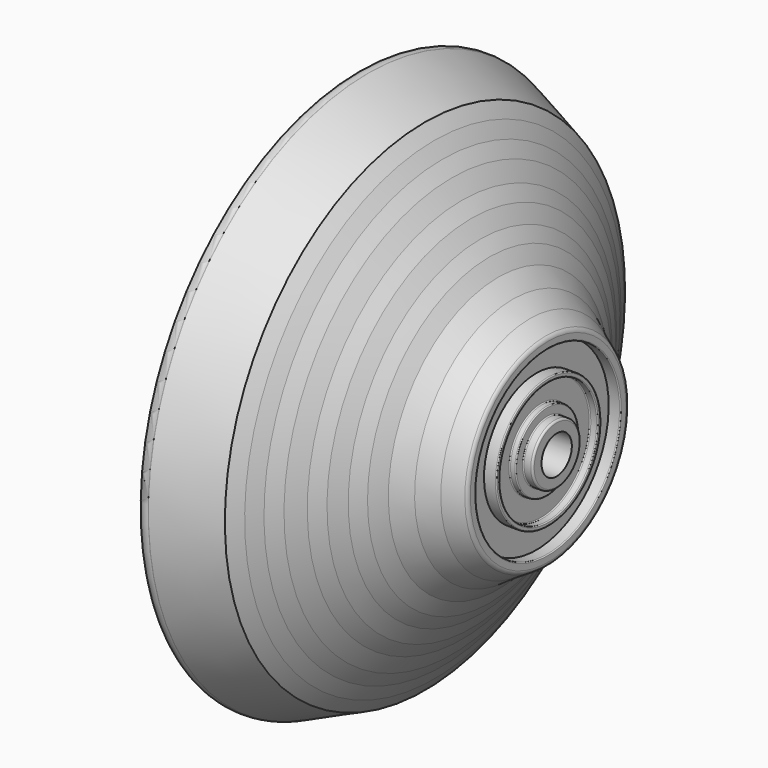
from build123d import *

# Parameters (mm, degrees)
F2_R = 0.1
F3_R = 0.2
F4_R = 0.5
F5_R = 0.5
F8_R = 0.85


with BuildPart() as f1:
    # F0 (on Front) → F1 (revolve)
    with BuildSketch(Plane.XZ):
        with BuildLine():
            Line((-4.2, 2), (-1.4, 2))
            Line((-1.4, 2), (-1.4, 3.17))
            Line((-1.4, 3.17), (-2.4, 3.17))
            Line((-2.4, 3.17), (-2.4, 4.15))
            Line((-2.4, 4.15), (-3.05, 4.15))
            Line((-3.05, 4.15), (-3.05, 6.45))
            Line((-3.05, 6.45), (-2.25, 6.45))
            Line((-2.25, 6.45), (-2.25, 6.9))
            Line((-2.25, 6.9), (-3.55, 6.9))
            Line((-3.55, 6.9), (-3.55, 9.55))
            Line((-3.55, 9.55), (-2.3, 9.55))
            Line((-2.3, 9.55), (-2.3, 10.55))
            Line((-2.3, 10.55), (-4.2488235049, 11.7284217849))
            Line((-4.2488235049, 11.7284217849), (-6.0193808361, 12.9681793751))
            Line((-6.0193808361, 12.9681793751), (-7.5602556007, 14.5090541396))
            Line((-7.5602556007, 14.5090541396), (-9.4593313096, 17.4266965415))
            Line((-9.4593313096, 17.4266965415), (-11.397791514, 20.4048472599))
            Line((-11.397791514, 20.4048472599), (-13.4484577999, 23.5553856402))
            Line((-13.4484577999, 23.5553856402), (-15.2898428789, 26.3843951207))
            Line((-15.2898428789, 26.3843951207), (-15.3, 26.4))
            Line((-15.3, 26.4), (-21.3, 26.4))
            Line((-21.3, 26.4), (-21.3, 28.9833333333))
            Line((-21.3, 28.9833333333), (-22.5, 29.5))
            Line((-22.5, 29.5), (-22.5, 24.5013962977))
            ThreePointArc((-22.5, 24.5013962977), (-21.9482556511, 23.6074908938), (-20.9018662575, 23.7))
            Line((-20.9018662575, 23.7), (-20.5080900341, 24.4))
            Line((-20.5080900341, 24.4), (-15.4300203026, 24.4))
            Line((-15.4300203026, 24.4), (-14.8718719174, 23.5424894817))
            Line((-14.8718719174, 23.5424894817), (-13.0431798353, 20.7329808699))
            Line((-13.0431798353, 20.7329808699), (-11.1785135129, 17.8682032825))
            Line((-11.1785135129, 17.8682032825), (-9.4125806174, 15.1551146623))
            Line((-9.4125806174, 15.1551146623), (-8.5412627086, 13.8106271625))
            Line((-8.5412627086, 13.8106271625), (-8.0127408728, 12.4712157995))
            Line((-8.0127408728, 12.4712157995), (-7.6767695136, 11.0429953784))
            Line((-7.6767695136, 11.0429953784), (-7.5, 9.6929371357))
            Line((-7.5, 9.6929371357), (-7.5, 8.5))
            Line((-7.5, 8.5), (-4.75, 8.5))
            Line((-4.75, 8.5), (-4.8163929872, 7.8235659748))
            Line((-4.8163929872, 7.8235659748), (-4.75, 7.1570291184))
            Line((-4.75, 7.1570291184), (-4.8163929872, 6.4776679501))
            Line((-4.8163929872, 6.4776679501), (-4.75, 5.7739662006))
            Line((-4.75, 5.7739662006), (-4.25, 5.7739662006))
            Line((-4.25, 5.7739662006), (-4.3176623901, 5.0816159641))
            Line((-4.3176623901, 5.0816159641), (-4.25, 4.4365157373))
            Line((-4.25, 4.4365157373), (-4.3095897044, 3.8267686403))
            Line((-4.3095897044, 3.8267686403), (-4.25, 3.17))
            Line((-4.25, 3.17), (-4.9999979152, 2.6389400014))
            Line((-4.9999979152, 2.6389400014), (-5.4533858784, 1.9280725392))
            Line((-5.4533858784, 1.9280725392), (-5.7284533243, 1.1602115126))
            Line((-5.7284533243, 1.1602115126), (-6.078645587, 0.5922464188))
            Line((-6.078645587, 0.5922464188), (-6.3, 0))
            Line((-6.3, 0), (-5.1852456548, 0))
            Line((-5.1852456548, 0), (-4.2, 2))
        make_face()
        Polygon((-9.4593313096, 17.4266965415), (-7.5602556007, 14.5090541396), (-8.4929022586, 16.0905005494), align=None)
        Polygon((-11.397791514, 20.4048472599), (-9.4593313096, 17.4266965415), (-10.4045527072, 19.0459996231), align=None)
        Polygon((-13.4484577999, 23.5553856402), (-11.397791514, 20.4048472599), (-12.4549735292, 22.1575423946), align=None)
        Polygon((-15.2898428789, 26.3843951207), (-13.4484577999, 23.5553856402), (-14.3121259439, 25.0234248466), align=None)
        Polygon((-10.3353289936, 16.4669086803), (-9.4125806174, 15.1551146623), (-11.1785135129, 17.8682032825), align=None)
        Polygon((-12.1445821899, 19.2208318679), (-11.1785135129, 17.8682032825), (-13.0431798353, 20.7329808699), align=None)
        Polygon((-14.0160004839, 22.095063141), (-13.0431798353, 20.7329808699), (-14.8718719174, 23.5424894817), align=None)
    revolve(axis=Axis((-5.7426228274, 0, 0), (-1, 0, 0)))

    # F2
    f2_edges = [f1.edges().sort_by_distance(p)[0] for p in [
        (-2.4, 0, -4.15),
        (-3.05, 0, -4.15),
        (-2.25, 0, -6.45),
        (-2.25, 0, -6.9),
        (-2.3, 0, -9.55),
        (-3.05, 0, -6.45),
        (-2.4, 0, -3.17),
    ]]
    fillet(f2_edges, radius=F2_R)

    # F3
    f3_edges = [f1.edges().sort_by_distance(p)[0] for p in [
        (-1.4, 0, -3.17),
    ]]
    fillet(f3_edges, radius=F3_R)

    # F4
    f4_edges = [f1.edges().sort_by_distance(p)[0] for p in [
        (-15.43002, 0, -24.4),
    ]]
    fillet(f4_edges, radius=F4_R)

    # F5
    f5_edges = [f1.edges().sort_by_distance(p)[0] for p in [
        (-2.3, 0, -10.55),
    ]]
    fillet(f5_edges, radius=F5_R)

    # F8
    f8_edges = [f1.edges().sort_by_distance(p)[0] for p in [
        (-22.5, 0, -29.5),
    ]]
    fillet(f8_edges, radius=F8_R)


with BuildPart() as f7:
    # F6 (on Front) → F7 (revolve)
    with BuildSketch(Plane.XZ):
        Polygon((-21.3, 28.9833333333), (-21.3, 26.4), (-15.3, 26.4), align=None)
    revolve(axis=Axis((-13.7036303058, 0, 0), (-1, 0, 0)))


solid = Compound([f1.part, f7.part])
